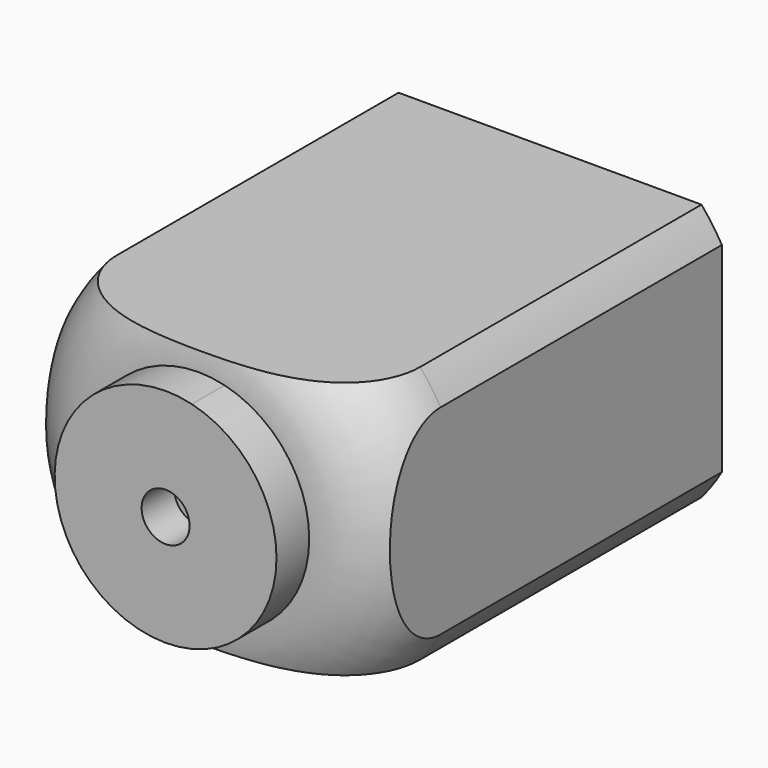
from build123d import *

# Parameters (mm, degrees)
F1_DEPTH    = 25.4
F2_T2_ANGLE = 136.8806858284
F2_T4_ANGLE = 136.8806858284
F2_T6_ANGLE = 136.8806858284
F2_T8_ANGLE = 136.8806858285
F3_R        = 1.3857299945
F4_DEPTH    = 2.3622
F5_R        = 2.5973758292
F5_R_2      = 1.5258073578
F6_DEPTH    = 2.54
F7_R        = 0.6147751451
F8_DEPTH    = 7.6708


# Not quite as in the source:
# - a fillet or chamfer that OpenCascade refuses, or shapes differently, is made with other operations: its cross-section is extruded or revolved along the edge and cut away or added
# - a feature names something its author has since deleted; it is built from what else it names


with BuildPart() as f1:
    # F0 (on Front) → F1 (new body)
    with BuildSketch(Plane.XZ):
        with BuildLine():
            Line((9.9314, -5.7745984882), (9.9314, 5.7745984882))
            ThreePointArc((9.9314, 5.7745984882), (9.3786903902, 6.6346710713), (8.7517057092, 7.4422))
            Line((8.7517057092, 7.4422), (-8.7517057092, 7.4422))
            ThreePointArc((-8.7517057092, 7.4422), (-9.3786903902, 6.6346710713), (-9.9314, 5.7745984882))
            Line((-9.9314, 5.7745984882), (-9.9314, -5.7745984882))
            ThreePointArc((-9.9314, -5.7745984882), (-9.3786903902, -6.6346710713), (-8.7517057092, -7.4422))
            Line((-8.7517057092, -7.4422), (8.7517057092, -7.4422))
            ThreePointArc((8.7517057092, -7.4422), (9.3786903902, -6.6346710713), (9.9314, -5.7745984882))
        make_face()
    extrude(amount=F1_DEPTH)

    # F2: fillet of radius 5.08 on 4 edges, made by hand

    # F2_s1 → F2_t2 (revolve, cut)
    with BuildSketch(Plane(origin=(0, 0, 0), x_dir=(0, 1, 0), z_dir=(0.9714801037, 0, -0.2371210832))):
        with BuildLine():
            ThreePointArc((-20.32, 11.4881980162), (-23.9121024484, 10.0003004647), (-25.4, 6.4081980162))
            Line((-25.4, 6.4081980162), (-25.4, 11.4881980162))
            Line((-25.4, 11.4881980162), (-20.32, 11.4881980162))
        make_face()
    revolve(axis=Axis((0, -25.4, 0), (0, -1, 0)), revolution_arc=F2_T2_ANGLE, mode=Mode.SUBTRACT)

    # F2_s3 → F2_t4 (revolve, cut)
    with BuildSketch(Plane(origin=(0, 0, 0), x_dir=(0, 1, 0), z_dir=(-0.5470373523, 0, -0.837108198))):
        with BuildLine():
            ThreePointArc((-20.32, 11.4881980162), (-23.9121024484, 10.0003004647), (-25.4, 6.4081980162))
            Line((-25.4, 6.4081980162), (-25.4, 11.4881980162))
            Line((-25.4, 11.4881980162), (-20.32, 11.4881980162))
        make_face()
    revolve(axis=Axis((0, -25.4, 0), (0, -1, 0)), revolution_arc=F2_T4_ANGLE, mode=Mode.SUBTRACT)

    # F2_s5 → F2_t6 (revolve, cut)
    with BuildSketch(Plane(origin=(0, 0, 0), x_dir=(0, 1, 0), z_dir=(0.5470373523, 0, 0.837108198))):
        with BuildLine():
            ThreePointArc((-20.32, 11.4881980162), (-23.9121024484, 10.0003004647), (-25.4, 6.4081980162))
            Line((-25.4, 6.4081980162), (-25.4, 11.4881980162))
            Line((-25.4, 11.4881980162), (-20.32, 11.4881980162))
        make_face()
    revolve(axis=Axis((0, -25.4, 0), (0, -1, 0)), revolution_arc=F2_T6_ANGLE, mode=Mode.SUBTRACT)

    # F2_s7 → F2_t8 (revolve, cut)
    with BuildSketch(Plane(origin=(0, 0, 0), x_dir=(0, 1, 0), z_dir=(-0.9714801037, 0, 0.2371210832))):
        with BuildLine():
            ThreePointArc((-20.32, 11.4881980162), (-23.9121024484, 10.0003004647), (-25.4, 6.4081980162))
            Line((-25.4, 6.4081980162), (-25.4, 11.4881980162))
            Line((-25.4, 11.4881980162), (-20.32, 11.4881980162))
        make_face()
    revolve(axis=Axis((0, -25.4, 0), (0, -1, 0)), revolution_arc=F2_T8_ANGLE, mode=Mode.SUBTRACT)

    # F3 (on face) → F4 (join)
    with BuildSketch(Plane.XZ.offset(25.4)):
        with BuildLine():
            ThreePointArc((1.5195188547, 6.2254368734), (-5.231499759, 3.7008663967), (-5.364355094, -3.5055236756))
            ThreePointArc((-5.364355094, -3.5055236756), (-2.3548191815, -5.9598513771), (1.5195188547, -6.2254368734))
            ThreePointArc((1.5195188547, -6.2254368734), (3.7008663967, -5.231499759), (5.364355094, -3.5055236756))
            ThreePointArc((5.364355094, -3.5055236756), (5.9598513771, 2.3548191815), (1.5195188547, 6.2254368734))
        make_face()
        Circle(F3_R, mode=Mode.SUBTRACT)
    extrude(amount=F4_DEPTH)

    # F5 (on face) → F6 (join)
    with BuildSketch(Plane.XZ):
        Circle(F5_R)
        Circle(F5_R_2, mode=Mode.SUBTRACT)
    extrude(amount=-F6_DEPTH)

    # F7 (on Front) → F8 (join)
    with BuildSketch(Plane.XZ):
        Circle(F7_R)
    extrude(amount=-F8_DEPTH)


solid = f1.part
